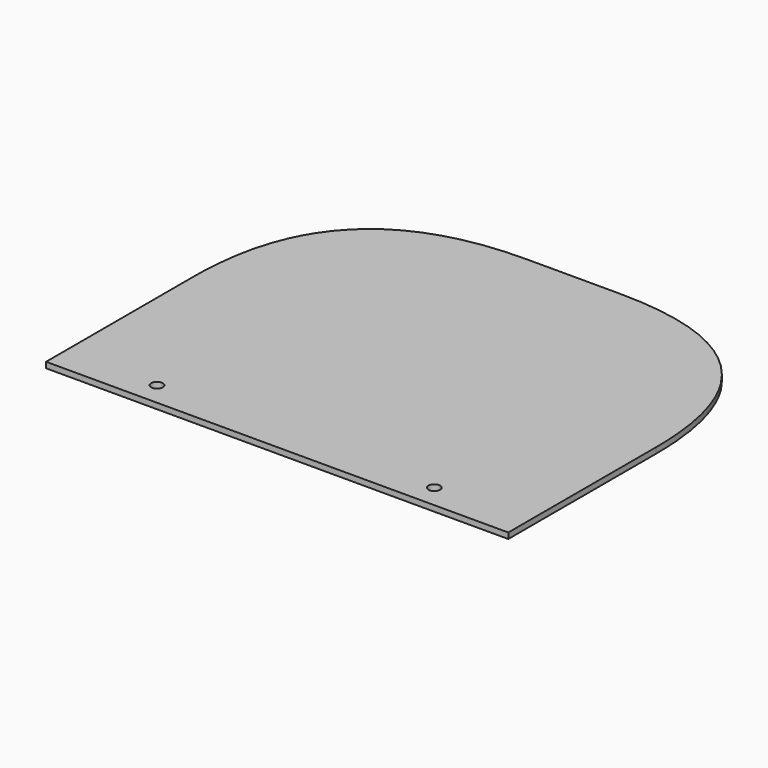
from build123d import *

# Parameters (mm, degrees)
F0_W        = 254
F0_H        = 203.2
F1_DEPTH    = 3.175
F2_T1_DEPTH = 511.175
F3_R        = 3.175
F4_DEPTH    = 3.175


# Not quite as in the source:
# - a fillet or chamfer that OpenCascade refuses, or shapes differently, is made with other operations: its cross-section is extruded or revolved along the edge and cut away or added


with BuildPart() as f1:
    # F0 (on Top) → F1 (new body)
    with BuildSketch(Plane.XY):
        with Locations((-9.1833584011, 11.7048747692)):
            Rectangle(F0_W, F0_H)
    extrude(amount=F1_DEPTH)

    # F2: fillet of radius 101.6 on 2 edges, made by hand

    # F2_s2 → F2_t1 (cut)
    with BuildSketch(Plane.XY.offset(-254)):
        with BuildLine():
            add(Edge.make_bspline(
                [(-136.1833584011, 11.7048747692), (-136.1833584011, 113.3048747692), (-34.5833584011, 113.3048747692)],
                knots=[0, 0, 0, 1, 1, 1], degree=2, weights=[1, 1, 1]))
            Line((-34.5833584011, 113.3048747692), (-136.1833584011, 113.3048747692))
            Line((-136.1833584011, 113.3048747692), (-136.1833584011, 11.7048747692))
        make_face()
        with BuildLine():
            add(Edge.make_bspline(
                [(117.8166415989, 11.7048747692), (117.8166415989, 113.3048747692), (16.2166415989, 113.3048747692)],
                knots=[0, 0, 0, 1, 1, 1], degree=2, weights=[1, 1, 1]))
            Line((16.2166415989, 113.3048747692), (117.8166415989, 113.3048747692))
            Line((117.8166415989, 113.3048747692), (117.8166415989, 11.7048747692))
        make_face()
    extrude(amount=F2_T1_DEPTH, mode=Mode.SUBTRACT)

    # F3 (on face) → F4 (cut)
    with BuildSketch(Plane.XY.offset(3.175)):
        with Locations((-85.3833584011, -77.1951252308)):
            Circle(F3_R)
        with Locations((67.0166415989, -77.1951252308)):
            Circle(F3_R)
    extrude(amount=-F4_DEPTH, mode=Mode.SUBTRACT)


solid = f1.part
